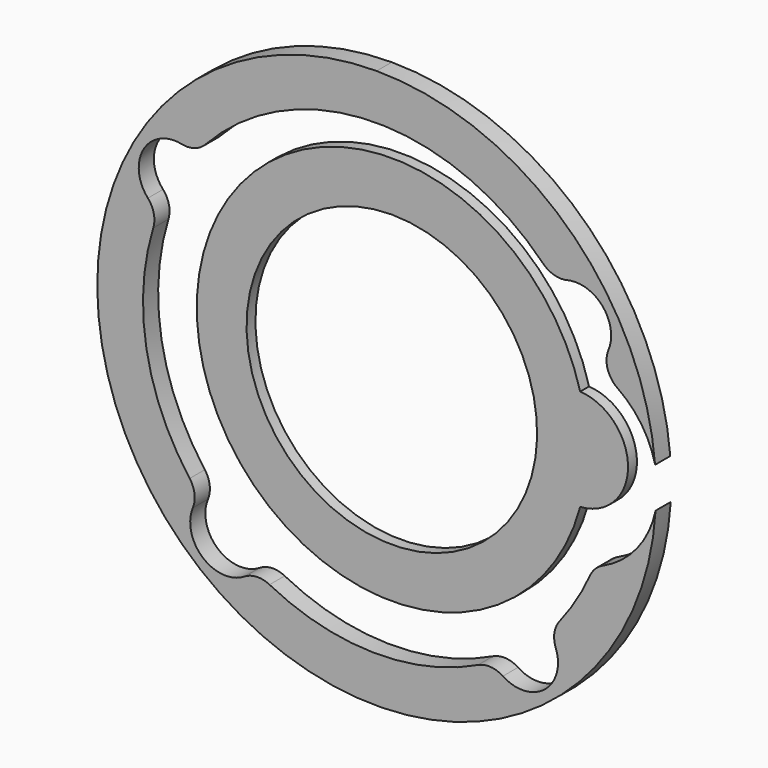
from build123d import *

# Parameters (mm, degrees)
F0_W           = 9.5
F0_H           = 9.8
F2_R           = 3.5
F3_DEPTH       = 25
F5_DEPTH       = 10
F7_SIZE        = 2
F8_DEPTH       = 25
F9_R           = 5
F10_DEPTH      = 6
F11_W          = 122.7332167327
F11_H          = 9.202274261
F11_W_2        = 118.1512214243
F11_H_2        = 11.7236196529
F12_DEPTH      = 75.5
F12_DEPTH_BACK = 118.2


# Not quite as in the source:
# - a feature names something its author has since deleted; it is built from what else it names


with BuildPart() as f1:
    # F0 (on Right) → F1 (revolve)
    with BuildSketch(Plane.YZ):
        Polygon((0, 15.2), (0, 28.6), (0, 38.4), (0, 55), (-3, 55), (-8, 55), (-8, 50), (-8, 39), (-8, 24.9987460632), (-8, 15.2), align=None)
        with Locations((4.75, 33.5)):
            Rectangle(F0_W, F0_H)
    revolve(axis=Axis((0, 5.6388881058, 0), (0, 1, 0)))

    # F2 (on face) → F3 (cut)
    with BuildSketch(Plane(origin=(0, 0, 0), x_dir=(-1, 0, 0), z_dir=(0, 1, 0))):
        with Locations((-28.6948903703, -35.9527921953)):
            Circle(F2_R)
        with Locations((39.8371685741, 23)):
            Circle(F2_R)
        with Locations((30.4043578574, -35.1233700587)):
            Circle(F2_R)
        with Locations((-39.5545513391, 23.3937592234)):
            Circle(F2_R)
    extrude(amount=-F3_DEPTH, mode=Mode.SUBTRACT)


with BuildPart() as f5:
    # F4 (on face) → F5 (new body)
    with BuildSketch(Plane(origin=(0, 9.5, 0), x_dir=(-1, 0, 0), z_dir=(0, 1, 0))):
        with BuildLine():
            ThreePointArc((-37.0795890411, -9.9831896979), (-38.4, 0), (-37.0795890411, 9.9831896979))
            ThreePointArc((-37.0795890411, 9.9831896979), (-46.5, 0), (-37.0795890411, -9.9831896979))
        make_face()
    extrude(amount=-F5_DEPTH)


with BuildPart() as f1_1:
    add(f1.part)

    # F6: union F5
    add(f5.part)

    # F7
    f7_edges = [f1_1.edges().sort_by_distance(p)[0] for p in [
        (-38.4, 9.5, 0),
        (46.5, 9.5, 0),
    ]]
    chamfer(f7_edges, length=F7_SIZE)

    # F2 (on face) → F8 (cut)
    with BuildSketch(Plane(origin=(0, 0, 0), x_dir=(-1, 0, 0), z_dir=(0, 1, 0))):
        with BuildLine():
            ThreePointArc((-32.758400191, 32.293764366), (-34.9517475646, 30.9945529981), (-37.5005356453, 30.9455407609))
            ThreePointArc((-37.5005356453, 30.9455407609), (-44.4666515342, 28.7024423136), (-45.6265051805, 21.4765859117))
            ThreePointArc((-45.6265051805, 21.4765859117), (-45.4543437959, 18.1543829003), (-47.4047637825, 15.4594739469))
            ThreePointArc((-47.4047637825, 15.4594739469), (-55.2129137143, -1.2460492891), (-44.5054093348, -16.2590790271))
            ThreePointArc((-44.5054093348, -16.2590790271), (-43.0175767772, -17.2873268137), (-41.9928754074, -18.7776040809))
            ThreePointArc((-41.9928754074, -18.7776040809), (-39.3121130623, -23.886351052), (-36.0129506984, -28.6193532771))
            ThreePointArc((-36.0129506984, -28.6193532771), (-34.9880846428, -30.9535281736), (-35.24718874, -33.4895857334))
            ThreePointArc((-35.24718874, -33.4895857334), (-33.0615041222, -41.4238692685), (-24.8400834669, -41.7957763419))
            ThreePointArc((-24.8400834669, -41.7957763419), (-22.424614561, -40.9807715296), (-19.9212921248, -41.4625387558))
            ThreePointArc((-19.9212921248, -41.4625387558), (0.6532544849, -45.9953612724), (21.0907724926, -40.8800601231))
            ThreePointArc((21.0907724926, -40.8800601231), (23.5794032698, -40.3273940989), (26.017043636, -41.0734720606))
            ThreePointArc((26.017043636, -41.0734720606), (34.224586227, -40.4682307198), (36.1840595318, -32.4750750957))
            ThreePointArc((36.1840595318, -32.4750750957), (35.8530371648, -29.9473988759), (36.8112004323, -27.585059774))
            ThreePointArc((36.8112004323, -27.585059774), (45.3165258085, -7.9001575079), (43.9739461252, 13.5015577685))
            ThreePointArc((43.9739461252, 13.5015577685), (43.8716778697, 16.0487648828), (45.038491918, 18.315319064))
            ThreePointArc((45.038491918, 18.315319064), (45.8993464006, 26.5), (38.3807775469, 29.8468186171))
            ThreePointArc((38.3807775469, 29.8468186171), (35.8344770228, 29.9696051004), (33.6796650808, 31.3317755649))
            ThreePointArc((33.6796650808, 31.3317755649), (0.6659863832, 45.9951786836), (-32.758400191, 32.293764366))
        make_face()
        with Locations((-28.6948903703, -35.9527921953)):
            Circle(F2_R, mode=Mode.SUBTRACT)
        with Locations((30.4043578574, -35.1233700587)):
            Circle(F2_R, mode=Mode.SUBTRACT)
        with Locations((-39.5545513391, 23.3937592234)):
            Circle(F2_R, mode=Mode.SUBTRACT)
        with Locations((39.8371685741, 23)):
            Circle(F2_R, mode=Mode.SUBTRACT)
    extrude(amount=-F8_DEPTH, mode=Mode.SUBTRACT)

    # F9 (on face) → F10 (cut)
    with BuildSketch(Plane.XZ.offset(8)):
        with Locations((-39.8371685741, 23)):
            Circle(F9_R)
        with Locations((28.6948903703, -35.9527921953)):
            Circle(F9_R)
    extrude(amount=-F10_DEPTH, mode=Mode.SUBTRACT)

    # F11 (on Top) → F12 (cut, two sides)
    with BuildSketch(Plane.XY) as f12_sk:
        with Locations((2.4499390274, -8.3294190699)):
            Rectangle(F11_W, F11_H)
        with Locations((1.2021679431, 8.0409679795)):
            Rectangle(F11_W_2, F11_H_2)
    extrude(amount=-F12_DEPTH, mode=Mode.SUBTRACT)
    extrude(f12_sk.sketch, amount=F12_DEPTH_BACK, mode=Mode.SUBTRACT)


solid = f1_1.part
